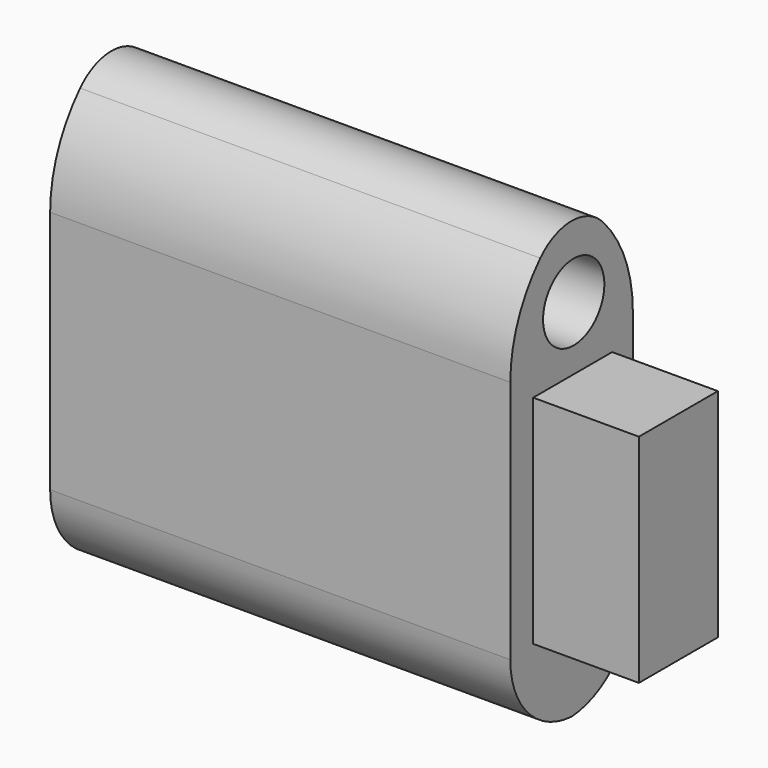
from build123d import *

# Parameters (mm, degrees)
F0_W        = 76.3128548861
F0_H        = 76.6920521855
F1_DEPTH    = 25.4
F2_T1_DEPTH = 189.756750182
F3_T1_DEPTH = 143.7659818188
F4_R        = 8.9325225018
F6_D        = 12.7
F7_W        = 16.36798447
F7_H        = 35.9481759369
F8_DEPTH    = 17.526


# Not quite as in the source:
# - a fillet or chamfer that OpenCascade refuses, or shapes differently, is made with other operations: its cross-section is extruded or revolved along the edge and cut away or added


with BuildPart() as f1:
    # F0 (on Front) → F1 (new body)
    with BuildSketch(Plane.XZ):
        with Locations((38.156427443, -38.3460260928)):
            Rectangle(F0_W, F0_H)
    extrude(amount=F1_DEPTH)

    # F2: fillet of radius 22.6887790592 on 2 edges, made by hand

    # F2_s2 → F2_t1 (cut)
    with BuildSketch(Plane.YZ.offset(-56.721947648)):
        with BuildLine():
            ThreePointArc((-2.7112209408, 0), (-18.7546104704, -6.6453895296), (-25.4, -22.6887790592))
            Line((-25.4, -22.6887790592), (-25.4, 0))
            Line((-25.4, 0), (-2.7112209408, 0))
        make_face()
        with BuildLine():
            ThreePointArc((-22.6887790592, 0), (-6.6453895296, -6.6453895296), (0, -22.6887790592))
            Line((0, -22.6887790592), (0, 0))
            Line((0, 0), (-22.6887790592, 0))
        make_face()
    extrude(amount=F2_T1_DEPTH, mode=Mode.SUBTRACT)

    # F3: fillet of radius 13.4906253865 on 2 edges, made by hand

    # F3_s2 → F3_t1 (cut)
    with BuildSketch(Plane.YZ.offset(-33.7265634664)):
        with BuildLine():
            ThreePointArc((-25.4, -63.201426799), (-21.4486873067, -72.7407394923), (-11.9093746135, -76.6920521855))
            Line((-11.9093746135, -76.6920521855), (-25.4, -76.6920521855))
            Line((-25.4, -76.6920521855), (-25.4, -63.201426799))
        make_face()
        with BuildLine():
            ThreePointArc((0, -63.201426799), (-3.9513126933, -72.7407394923), (-13.4906253865, -76.6920521855))
            Line((-13.4906253865, -76.6920521855), (0, -76.6920521855))
            Line((0, -76.6920521855), (0, -63.201426799))
        make_face()
    extrude(amount=F3_T1_DEPTH, mode=Mode.SUBTRACT)

    # F4
    f4_edges = [f1.edges().sort_by_distance(p)[0] for p in [
        (38.156427, -12.7, -2.317108),
    ]]
    fillet(f4_edges, radius=F4_R)

    # F6 (through all)
    with Locations(Plane.YZ.offset(76.3128548861)):
        with Locations((-12.2666405514, -16.3046810776)):
            Hole(F6_D / 2)

    # F7 (on face) → F8 (join)
    with BuildSketch(Plane.YZ.offset(76.3128548861)):
        with Locations((-12.4732137192, -44.8362212628)):
            Rectangle(F7_W, F7_H)
    extrude(amount=F8_DEPTH)


solid = f1.part
